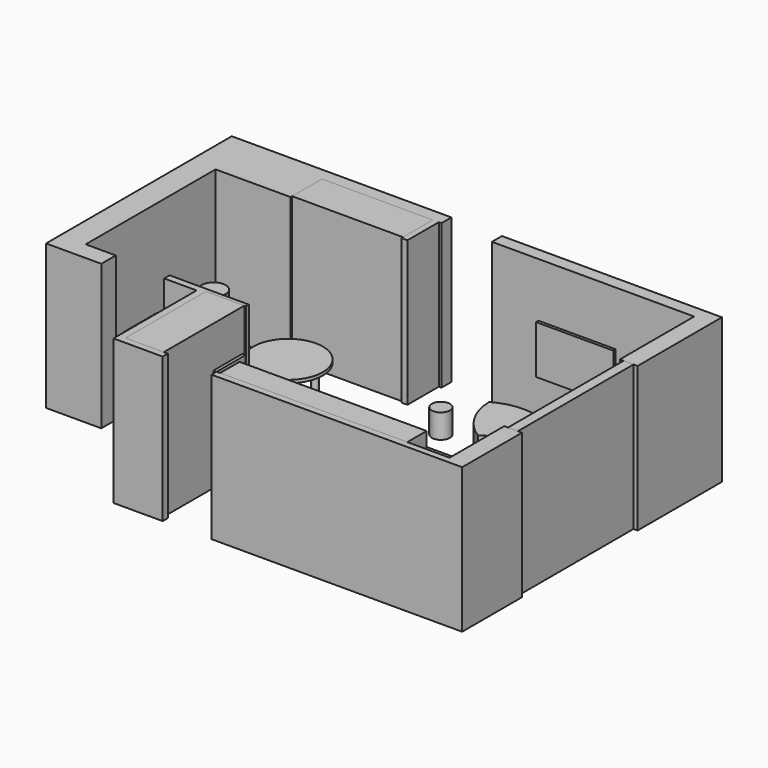
from build123d import *

# Parameters (mm, degrees)
F1_DEPTH  = 2400
F0_W      = 537.1888577938
F0_H      = 112.3662590981
F0_W_2    = 53.346157074
F0_H_2    = 600
F0_W_3    = 1250
F0_H_3    = 430
F0_W_4    = 550
F0_H_4    = 500
F0_W_5    = 600
F0_H_5    = 1400
F2_DEPTH  = 900
F3_W      = 3100
F3_H      = 400
F4_DEPTH  = 800
F0_H_6    = 650
F5_DEPTH  = 1900
F0_W_6    = 2100
F0_H_7    = 250
F6_DEPTH  = 900
F7_DEPTH  = 450
F0_W_7    = 350
F0_H_8    = 350
F8_DEPTH  = 910
F9_DEPTH  = 750
F10_DEPTH = 910
F0_W_8    = 164.1221046448
F0_H_9    = 2394.7671353817
F11_DEPTH = 2400
F0_R      = 575
F0_R_2    = 50
F12_DEPTH = 750
F13_DEPTH = 700
F0_W_9    = 1280
F0_H_10   = 50
F15_DEPTH = 1500
F16_W     = 1280
F16_H     = 700
F17_DEPTH = 50
F18_DEPTH = 400
F0_R_3    = 150
F0_H_11   = 400
F19_DEPTH = 1600
F20_W     = 580
F20_H     = 540
F20_H_2   = 500
F21_DEPTH = 380
F22_W     = 600
F22_H     = 600
F23_DEPTH = 25
F22_W_2   = 2500
F22_H_2   = 100
F24_DEPTH = 30
F25_W     = 10
F25_H     = 800
F26_DEPTH = 10
F27_W     = 700
F27_H     = 600
F28_DEPTH = 60
F0_W_10   = 1835.4965090752
F0_H_12   = 616.584777832
F29_DEPTH = 2400
F0_R_4    = 200
F30_DEPTH = 1000


# Not quite as in the source:
# - a feature names something its author has since deleted; it is built from what else it names


with BuildPart() as f1:
    # F0 (on Top) → F1 (new body)
    with BuildSketch(Plane.XY):
        Polygon((5332.8738090396, 2704.7533988953), (5394.4396972656, 2704.7533988953), (5558.5618019104, 2704.7533988953), (5626.5387535095, 2704.7533988953), (5626.5387535095, 4450.9944915771), (5332.8738090396, 4450.9944915771), (5332.8738090396, 4243.6318397522), align=None)
        Polygon((4032.8738090396, 4243.6318397522), (5332.8738090396, 4243.6318397522), (5332.8738090396, 4450.9944915771), (1981.1851978302, 4450.9944915771), (1981.1851978302, 4243.6318397522), (2752.8738090396, 4243.6318397522), align=None)
    extrude(amount=F1_DEPTH)


with BuildPart() as f1b:
    # F0 (on Top) → F1, piece 2 (new body)
    with BuildSketch(Plane.XY):
        Polygon((5332.8738090396, 309.9862635136), (5332.8738090396, -822.1663832664), (4632.8738090396, -822.1663832664), (1532.8738090396, -822.1663832664), (1474.7484922409, -822.1663832664), (1474.7484922409, -928.7706017494), (5626.5387535095, -928.7706017494), (5626.5387535095, 309.9862635136), (5558.5618019104, 309.9862635136), (5394.4396972656, 309.9862635136), align=None)
    extrude(amount=F1_DEPTH)


with BuildPart() as f1c:
    # F0 (on Top) → F1, piece 3 (new body)
    with BuildSketch(Plane.XY):
        Polygon((597.9725122452, -822.1663832664), (-37.1261909604, -822.1663832664), (-37.1261909604, -26.347534731), (-37.1261909604, 845.5312275887), (-37.1261909604, 905.5312275887), (-150.5666673183, 905.5312275887), (-150.5666673183, 793.1649684906), (-150.5666673183, -928.7706017494), (664.8011207581, -928.7706017494), (664.8011207581, -822.1663832664), align=None)
        with Locations((-419.1610962152, 849.3480980396)):
            Rectangle(F0_W, F0_H)
        Polygon((-37.1261909604, 845.5312275887), (597.9725122452, 845.5312275887), (624.0934729576, 845.5312275887), (624.0934729576, 905.5312275887), (597.9725122452, 905.5312275887), (-37.1261909604, 905.5312275887), align=None)
    extrude(amount=F1_DEPTH)


with BuildPart() as f1d:
    # F0 (on Top) → F1, piece 4 (new body)
    with BuildSketch(Plane.XY):
        with Locations((1448.0754137039, -522.1663832664)):
            Rectangle(F0_W_2, F0_H_2)
    extrude(amount=F1_DEPTH)


with BuildPart() as f1e:
    # F0 (on Top) → F1, piece 5 (new body)
    with BuildSketch(Plane.XY):
        Polygon((1101.2586355209, 4243.6318397522), (1145.4427242279, 4243.6318397522), (1145.4427242279, 4450.9944915771), (-2494.3199157715, 4450.9944915771), (-2494.3199157715, 605.3053736687), (-1579.2272090912, 605.3053736687), (-1579.2272090912, 905.5312275887), (-2078.3698558807, 905.5312275887), (-2078.3698558807, 3594.8448181152), (-834.2378735542, 3594.8448181152), (-834.2378735542, 3627.0470619202), (-834.2378735542, 4243.6318397522), (1001.2586355209, 4243.6318397522), align=None)
        Polygon((1101.2586355209, 3594.8448181152), (1101.2586355209, 4243.6318397522), (1001.2586355209, 4243.6318397522), (1001.2586355209, 3627.0470619202), (1001.2586355209, 3594.8448181152), align=None)
    extrude(amount=F1_DEPTH)


with BuildPart() as f2:
    # F0 (on Top) → F2 (new body)
    with BuildSketch(Plane.XY):
        Polygon((1532.8738090396, -822.1663832664), (4632.8738090396, -822.1663832664), (4632.8738090396, -222.1663832664), (2132.8738090396, -222.1663832664), (1532.8738090396, -222.1663832664), align=None)
        with Locations((2757.8738090396, -517.1663832664)):
            Rectangle(F0_W_3, F0_H_3, mode=Mode.SUBTRACT)
        with Locations((3957.8738090396, -522.1663832664)):
            Rectangle(F0_W_4, F0_H_4, mode=Mode.SUBTRACT)
        with Locations((1832.8738090396, 477.8336167336)):
            Rectangle(F0_W_5, F0_H_5)
    extrude(amount=F2_DEPTH)

    # F0 (on Top) → F8 (join)
    with BuildSketch(Plane.XY):
        with Locations((2757.8738090396, -517.1663832664)):
            Rectangle(F0_W_3, F0_H_3)
        with Locations((2757.8738090396, -507.1663832664)):
            Rectangle(F0_W_7, F0_H_8, mode=Mode.SUBTRACT)
        with Locations((3157.8738090396, -507.1663832664)):
            Rectangle(F0_W_7, F0_H_8, mode=Mode.SUBTRACT)
    extrude(amount=F8_DEPTH)

    # F0 (on Top) → F9 (join)
    with BuildSketch(Plane.XY):
        with Locations((3157.8738090396, -507.1663832664)):
            Rectangle(F0_W_7, F0_H_8)
        with Locations((2757.8738090396, -507.1663832664)):
            Rectangle(F0_W_7, F0_H_8)
    extrude(amount=F9_DEPTH)

    # F0 (on Top) → F10 (join)
    with BuildSketch(Plane.XY):
        with Locations((3957.8738090396, -522.1663832664)):
            Rectangle(F0_W_4, F0_H_4)
    extrude(amount=F10_DEPTH)

    # F22 (on face) → F23 (join)
    with BuildSketch(Plane(origin=(0, -222.1663832664, 0), x_dir=(-1, 0, 0), z_dir=(0, 1, 0))):
        with Locations((-3607.9814311862, 500)):
            Rectangle(F22_W, F22_H)
        with Locations((-2807.9814311862, 500)):
            Rectangle(F22_W, F22_H)
    extrude(amount=F23_DEPTH)

    # F22 (on face) → F24 (cut)
    with BuildSketch(Plane(origin=(0, -222.1663832664, 0), x_dir=(-1, 0, 0), z_dir=(0, 1, 0))):
        with Locations((-3382.8738090396, 50)):
            Rectangle(F22_W_2, F22_H_2)
    extrude(amount=-F24_DEPTH, mode=Mode.SUBTRACT)


with BuildPart() as f4:
    # F3 (on face) → F4 (new body)
    with BuildSketch(Plane.XY.offset(2400)):
        with Locations((3082.8738090396, -622.1663832664)):
            Rectangle(F3_W, F3_H)
    extrude(amount=-F4_DEPTH)

    # F25 (on face) → F26 (cut)
    with BuildSketch(Plane(origin=(0, -422.1663832664, 0), x_dir=(-1, 0, 0), z_dir=(0, 1, 0))):
        with Locations((-2037.8738090396, 2000)):
            Rectangle(F25_W, F25_H)
        with Locations((-2547.8738090396, 2000)):
            Rectangle(F25_W, F25_H)
        with Locations((-3057.8738090396, 2000)):
            Rectangle(F25_W, F25_H)
        with Locations((-3567.8738090396, 2000)):
            Rectangle(F25_W, F25_H)
        with Locations((-4077.8738090396, 2000)):
            Rectangle(F25_W, F25_H)
    extrude(amount=-F26_DEPTH, mode=Mode.SUBTRACT)


with BuildPart() as f5:
    # F0 (on Top) → F5 (new body)
    with BuildSketch(Plane.XY):
        with Locations((5006.0084342957, -436.6334557533)):
            Rectangle(F0_W_5, F0_H_6)
    extrude(amount=F5_DEPTH)


with BuildPart() as f6:
    # F0 (on Top) → F6 (new body)
    with BuildSketch(Plane.XY):
        with Locations((3844.4396972656, 1352.8336167336)):
            Rectangle(F0_W_6, F0_H_7)
    extrude(amount=F6_DEPTH)

    # F0 (on Top) → F7 (join)
    with BuildSketch(Plane.XY):
        Polygon((2794.4396972656, 1477.8336167336), (4894.4396972656, 1477.8336167336), (4894.4396972656, 2727.8336167336), (4094.4396972656, 2727.8336167336), (4094.4396972656, 2087.8336167336), (2794.4396972656, 2087.8336167336), align=None)
    extrude(amount=F7_DEPTH)


with BuildPart() as f11:
    # F0 (on Top) → F11 (new body)
    with BuildSketch(Plane.XY):
        with Locations((5476.500749588, 1507.3698312044)):
            Rectangle(F0_W_8, F0_H_9)
    extrude(amount=F11_DEPTH)


with BuildPart() as f12:
    # F0 (on Top) → F12 (new body)
    with BuildSketch(Plane.XY):
        with Locations((0, 2500.5469322205)):
            Circle(F0_R)
        with Locations((-247.4873734153, 2253.0595588052)):
            Circle(F0_R_2, mode=Mode.SUBTRACT)
        with Locations((247.4873734153, 2253.0595588052)):
            Circle(F0_R_2, mode=Mode.SUBTRACT)
        with Locations((-247.4873734153, 2748.0343056358)):
            Circle(F0_R_2, mode=Mode.SUBTRACT)
        with Locations((247.4873734153, 2748.0343056358)):
            Circle(F0_R_2, mode=Mode.SUBTRACT)
        with Locations((247.4873734153, 2748.0343056358)):
            Circle(F0_R_2)
        with Locations((247.4873734153, 2253.0595588052)):
            Circle(F0_R_2)
        with Locations((-247.4873734153, 2748.0343056358)):
            Circle(F0_R_2)
        with Locations((-247.4873734153, 2253.0595588052)):
            Circle(F0_R_2)
    extrude(amount=F12_DEPTH)


with BuildPart() as f13:
    # F0 (on Top) → F13 (new body)
    with BuildSketch(Plane.XY):
        with Locations((0, 2500.5469322205)):
            Circle(F0_R)
        with Locations((-247.4873734153, 2253.0595588052)):
            Circle(F0_R_2, mode=Mode.SUBTRACT)
        with Locations((247.4873734153, 2253.0595588052)):
            Circle(F0_R_2, mode=Mode.SUBTRACT)
        with Locations((-247.4873734153, 2748.0343056358)):
            Circle(F0_R_2, mode=Mode.SUBTRACT)
        with Locations((247.4873734153, 2748.0343056358)):
            Circle(F0_R_2, mode=Mode.SUBTRACT)
    extrude(amount=F13_DEPTH)


with BuildPart() as f12_1:
    add(f12.part)

    # F14: cut F13
    add(f13.part, mode=Mode.SUBTRACT)


with BuildPart() as f15:
    # F0 (on Top) → F15 (new body)
    with BuildSketch(Plane.XY):
        with Locations((3392.8738090396, 4218.6318397522)):
            Rectangle(F0_W_9, F0_H_10)
    extrude(amount=F15_DEPTH)

    # F16 (on face) → F17 (cut)
    with BuildSketch(Plane.XZ.offset(-4193.6318397522)):
        with Locations((3392.8738090396, 350)):
            Rectangle(F16_W, F16_H)
    extrude(amount=-F17_DEPTH, mode=Mode.SUBTRACT)


with BuildPart() as f18:
    # F0 (on Top) → F18 (new body)
    with BuildSketch(Plane.XY):
        with BuildLine():
            ThreePointArc((2356.5598369582, 3718.6318397522), (2490.1661397403, 3245.7694746289), (2832.8738090396, 2893.6318397522))
            ThreePointArc((2832.8738090396, 2893.6318397522), (3175.5814783389, 3245.7694746289), (3309.187781121, 3718.6318397522))
            ThreePointArc((3309.187781121, 3718.6318397522), (2832.8738090396, 3839.3565699987), (2356.5598369582, 3718.6318397522))
        make_face()
    extrude(amount=F18_DEPTH)


with BuildPart() as f18b:
    # F0 (on Top) → F18, piece 2 (new body)
    with BuildSketch(Plane.XY):
        with Locations((4030.5371284485, 3705.1014900208)):
            Circle(F0_R_3)
    extrude(amount=F18_DEPTH)


with BuildPart() as f18c:
    # F0 (on Top) → F18, piece 3 (new body)
    with BuildSketch(Plane.XY):
        with Locations((1959.0933322906, 3213.9573097229)):
            Circle(F0_R_3)
    extrude(amount=F18_DEPTH)


with BuildPart() as f19:
    # F0 (on Top) → F19 (new body)
    with BuildSketch(Plane.XY):
        with Locations((5001.082611084, 4008.5523605347)):
            Rectangle(F0_W_5, F0_H_11)
    extrude(amount=F19_DEPTH)

    # F20 (on face) → F21 (cut)
    with BuildSketch(Plane.XZ.offset(-3808.5523605347)):
        with Locations((5001.082611084, 1320)):
            Rectangle(F20_W, F20_H)
        with Locations((5001.082611084, 780)):
            Rectangle(F20_W, F20_H_2)
        with Locations((5001.082611084, 260)):
            Rectangle(F20_W, F20_H_2)
    extrude(amount=-F21_DEPTH, mode=Mode.SUBTRACT)


with BuildPart() as f28:
    # F27 (on face) → F28 (new body)
    with BuildSketch(Plane.YZ.offset(-2078.3698558807)):
        with Locations((2026.7077445984, 500)):
            Rectangle(F27_W, F27_H)
    extrude(amount=F28_DEPTH)


with BuildPart() as f29:
    # F0 (on Top) → F29 (new body)
    with BuildSketch(Plane.XY):
        with Locations((83.5103809834, 3935.3394508362)):
            Rectangle(F0_W_10, F0_H_12)
    extrude(amount=F29_DEPTH)


with BuildPart() as f29b:
    # F0 (on Top) → F29, piece 2 (new body)
    with BuildSketch(Plane.XY):
        Polygon((-37.1261909604, -26.347534731), (-37.1261909604, -822.1663832664), (597.9725122452, -822.1663832664), (597.9725122452, 845.5312275887), (-37.1261909604, 845.5312275887), align=None)
    extrude(amount=F29_DEPTH)


with BuildPart() as f30:
    # F0 (on Top) → F30 (new body)
    with BuildSketch(Plane.XY):
        with Locations((-1673.9757061005, 3049.9031543732)):
            Circle(F0_R_4)
    extrude(amount=F30_DEPTH)


solid = Compound([f1.part, f1b.part, f1c.part, f1d.part, f1e.part, f2.part, f4.part, f5.part, f6.part, f11.part, f12_1.part, f15.part, f18.part, f18b.part, f18c.part, f19.part, f28.part, f29.part, f29b.part, f30.part])
